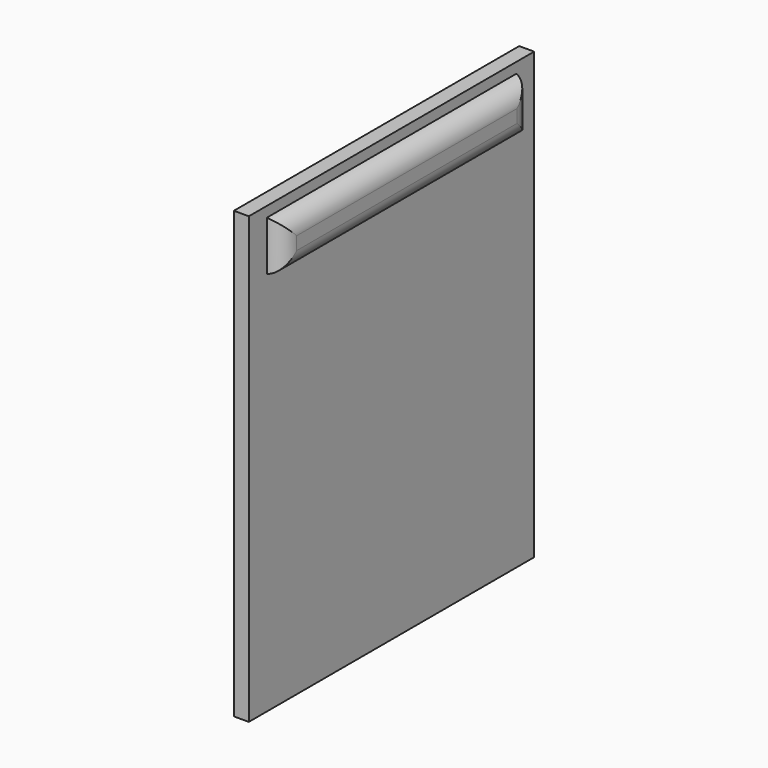
from build123d import *

# Parameters (mm, degrees)
F0_W        = 4.0632686578
F0_H        = 96.9379618764
F1_DEPTH    = 121
F2_W        = 94.1168889403
F2_H        = 118.3094680309
F3_DEPTH    = 0.2
F4_W        = 84.7520232201
F4_H        = 13.4229809046
F5_DEPTH    = 4.2
F6_T1_DEPTH = 109.4299485786
F6_T3_DEPTH = 38.1009062631


# Not quite as in the source:
# - a fillet or chamfer that OpenCascade refuses, or shapes differently, is made with other operations: its cross-section is extruded or revolved along the edge and cut away or added


with BuildPart() as f1:
    # F0 (on Top) → F1 (new body)
    with BuildSketch(Plane.XY):
        Rectangle(F0_W, F0_H)
    extrude(amount=F1_DEPTH)

    # F2 (on face) → F3 (join)
    with BuildSketch(Plane(origin=(-2.0316343289, 0, 0), x_dir=(0, -1, 0), z_dir=(-1, 0, 0))):
        with Locations((0, 60.4219585657)):
            Rectangle(F2_W, F2_H)
    extrude(amount=F3_DEPTH)

    # F4 (on face) → F5 (join)
    with BuildSketch(Plane.YZ.offset(2.0316343289)):
        with Locations((0, 111.4604696631)):
            Rectangle(F4_W, F4_H)
    extrude(amount=F5_DEPTH)

    # F6: fillet of radius 5 on 4 edges, made by hand

    # F6_s2 → F6_t1 (cut)
    with BuildSketch(Plane.XZ.offset(-54.7149742893)):
        with BuildLine():
            ThreePointArc((2.0316343289, 118.1719601154), (5.0395208818, 116.4767453929), (6.2316343289, 113.2363750437))
            Line((6.2316343289, 113.2363750437), (6.2316343289, 118.1719601154))
            Line((6.2316343289, 118.1719601154), (2.0316343289, 118.1719601154))
        make_face()
        with BuildLine():
            ThreePointArc((2.0316343289, 104.7489792109), (5.0395208818, 106.4441939334), (6.2316343289, 109.6845642826))
            Line((6.2316343289, 109.6845642826), (6.2316343289, 104.7489792109))
            Line((6.2316343289, 104.7489792109), (2.0316343289, 104.7489792109))
        make_face()
    extrude(amount=F6_T1_DEPTH, mode=Mode.SUBTRACT)

    # F6_s4 → F6_t3 (cut)
    with BuildSketch(Plane.XY.offset(92.4100165316)):
        with BuildLine():
            ThreePointArc((2.0316343289, -42.37601161), (5.0395208818, -40.6807968875), (6.2316343289, -37.4404265383))
            Line((6.2316343289, -37.4404265383), (6.2316343289, -42.37601161))
            Line((6.2316343289, -42.37601161), (2.0316343289, -42.37601161))
        make_face()
        with BuildLine():
            ThreePointArc((2.0316343289, 42.37601161), (5.0395208818, 40.6807968875), (6.2316343289, 37.4404265383))
            Line((6.2316343289, 37.4404265383), (6.2316343289, 42.37601161))
            Line((6.2316343289, 42.37601161), (2.0316343289, 42.37601161))
        make_face()
    extrude(amount=F6_T3_DEPTH, mode=Mode.SUBTRACT)


solid = f1.part
